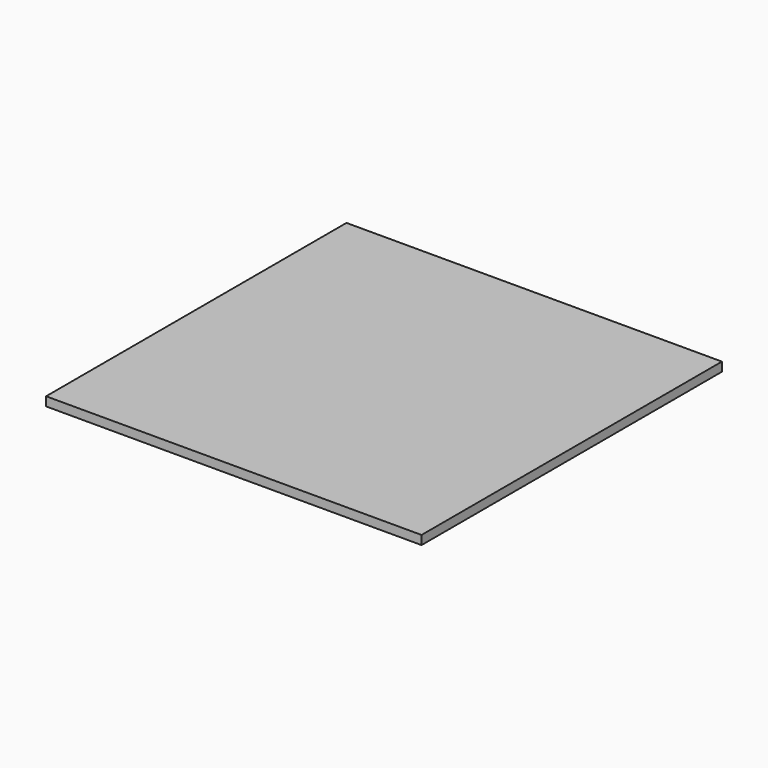
from build123d import *

# Parameters (mm, degrees)
F0_W     = 133.35
F0_H     = 133.35
F1_DEPTH = 3.175


# Not quite as in the source:
# - a feature of the source that left no trace in its solid (it failed there, or was rolled back) is left out


with BuildPart() as f1:
    # F0 (on Top) → F1 (new body)
    with BuildSketch(Plane.XY):
        Rectangle(F0_W, F0_H)
    extrude(amount=F1_DEPTH)


solid = f1.part
